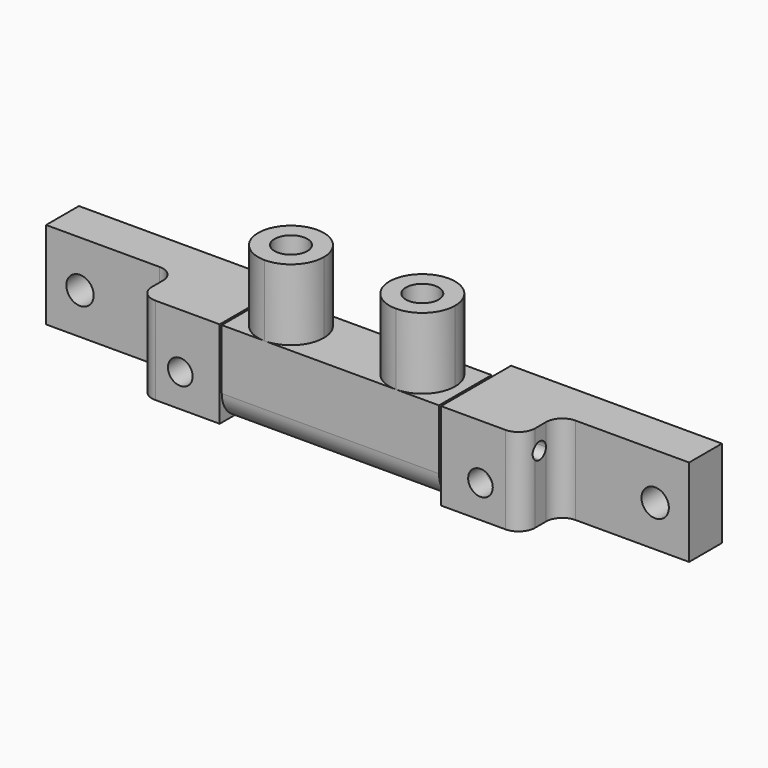
from build123d import *

# Parameters (mm, degrees)
F0_W     = 23.75
F0_H     = 3.5
F1_DEPTH = 16
F0_R     = 3
F2_DEPTH = 29
F3_R     = 2.25
F3_R_2   = 2.5
F4_DEPTH = 12.5
F5_R     = 3
F5_2_R   = 3
F7_DEPTH = 40
F8_R     = 5


with BuildPart() as f1:
    # F0 (on Top) → F1 (new body)
    with BuildSketch(Plane.XY):
        with Locations((-46.875, 6.25)):
            Rectangle(F0_W, F0_H)
        Polygon((-20.2244706452, -4), (-20.2244706452, 8), (-35, 8), (-35, 4.5), (-35, -4), align=None)
        Polygon((-35, 8), (-20.2244706452, 8), (-20.2244706452, 12), (-58.75, 12), (-58.75, 8), align=None)
    extrude(amount=F1_DEPTH)


with BuildPart() as f1b:
    # F0 (on Top) → F1, piece 2 (new body)
    with BuildSketch(Plane.XY):
        with BuildLine():
            ThreePointArc((-12, -4), (-18, 2.0000000001), (-11.9999999997, 8))
            Line((-11.9999999997, 8), (-19.8490470648, 8))
            Line((-19.8490470648, 8), (-19.8490470648, -4))
            Line((-19.8490470648, -4), (-12, -4))
        make_face()
        with BuildLine():
            ThreePointArc((-6, 2), (-7.7573593128, 6.242640687), (-11.9999999997, 8))
            ThreePointArc((-11.9999999997, 8), (-18, 2.0000000001), (-12, -4))
            ThreePointArc((-12, -4), (-7.7573593129, -2.2426406871), (-6, 2))
        make_face()
        with Locations((-12, 2)):
            Circle(F0_R, mode=Mode.SUBTRACT)
        with Locations((-12, 2)):
            Circle(F0_R)
        with BuildLine():
            ThreePointArc((12, -4), (6, 2.0000000207), (12.0000000413, 8))
            Line((12.0000000413, 8), (-11.9999999997, 8))
            ThreePointArc((-11.9999999997, 8), (-7.7573593128, 6.242640687), (-6, 2))
            ThreePointArc((-6, 2), (-7.7573593129, -2.2426406871), (-12, -4))
            Line((-12, -4), (12, -4))
        make_face()
        with BuildLine():
            ThreePointArc((18, 2), (17.8620020617, 3.2794263668), (17.4543560573, 4.5))
            ThreePointArc((17.4543560573, 4.5), (15.2403703666, 7.049752458), (12.0000000413, 8))
            ThreePointArc((12.0000000413, 8), (6, 2.0000000207), (12, -4))
            ThreePointArc((12, -4), (16.2426406871, -2.2426406871), (18, 2))
        make_face()
        with BuildLine():
            ThreePointArc((13.6583123952, 4.5), (14.6433820369, 3.4186371655), (15, 2))
            ThreePointArc((15, 2), (9.3566179631, 0.5813628345), (13.6583123952, 4.5))
        make_face(mode=Mode.SUBTRACT)
        with BuildLine():
            ThreePointArc((13.6583123952, 4.5), (9.3566179631, 0.5813628345), (15, 2))
            ThreePointArc((15, 2), (14.6433820369, 3.4186371655), (13.6583123952, 4.5))
        make_face()
        with BuildLine():
            ThreePointArc((12.0000000413, 8), (15.2403703666, 7.049752458), (17.4543560573, 4.5))
            ThreePointArc((17.4543560573, 4.5), (17.8620020617, 3.2794263668), (18, 2))
            ThreePointArc((18, 2), (16.2426406871, -2.2426406871), (12, -4))
            Line((12, -4), (19.8490470648, -4))
            Line((19.8490470648, -4), (19.8490470648, 8))
            Line((19.8490470648, 8), (12.0000000413, 8))
        make_face()
    extrude(amount=F1_DEPTH)

    # F0 (on Top) → F2 (join)
    with BuildSketch(Plane.XY):
        with BuildLine():
            ThreePointArc((-6, 2), (-7.7573593128, 6.242640687), (-11.9999999997, 8))
            ThreePointArc((-11.9999999997, 8), (-18, 2.0000000001), (-12, -4))
            ThreePointArc((-12, -4), (-7.7573593129, -2.2426406871), (-6, 2))
        make_face()
        with Locations((-12, 2)):
            Circle(F0_R, mode=Mode.SUBTRACT)
        with BuildLine():
            ThreePointArc((18, 2), (17.8620020617, 3.2794263668), (17.4543560573, 4.5))
            ThreePointArc((17.4543560573, 4.5), (15.2403703666, 7.049752458), (12.0000000413, 8))
            ThreePointArc((12.0000000413, 8), (6, 2.0000000207), (12, -4))
            ThreePointArc((12, -4), (16.2426406871, -2.2426406871), (18, 2))
        make_face()
        with BuildLine():
            ThreePointArc((13.6583123952, 4.5), (14.6433820369, 3.4186371655), (15, 2))
            ThreePointArc((15, 2), (9.3566179631, 0.5813628345), (13.6583123952, 4.5))
        make_face(mode=Mode.SUBTRACT)
    extrude(amount=F2_DEPTH)


with BuildPart() as f1c:
    # F0 (on Top) → F1, piece 3 (new body)
    with BuildSketch(Plane.XY):
        Polygon((35, 8), (20.2244706452, 8), (20.2244706452, -4), (35, -4), (35, 4.5), align=None)
        with Locations((46.875, 6.25)):
            Rectangle(F0_W, F0_H)
        Polygon((20.2244706452, 12), (20.2244706452, 8), (35, 8), (58.75, 8), (58.75, 12), align=None)
    extrude(amount=F1_DEPTH)


with BuildPart() as f4_tool:
    # F3 (on Front) → F4 (new body, symmetric)
    with BuildSketch(Plane.XZ):
        with Locations((-27.4271778762, 6)):
            Circle(F3_R)
        with Locations((27.4271778762, 6)):
            Circle(F3_R)
        with Locations((-52.55, 7.5)):
            Circle(F3_R_2)
        with Locations((52.55, 7.5)):
            Circle(F3_R_2)
    extrude(amount=F4_DEPTH, both=True)


with BuildPart() as f1_1:
    add(f1.part)

    # F4: cut by f4_tool
    add(f4_tool.part, mode=Mode.SUBTRACT)

    # F5
    f5_edges = [f1_1.edges().sort_by_distance(p)[0] for p in [
        (-35, -4, 8),
        (-35, 4.5, 8),
    ]]
    fillet(f5_edges, radius=F5_R)


with BuildPart() as f1c_1:
    add(f1c.part)

    # F4: cut by f4_tool
    add(f4_tool.part, mode=Mode.SUBTRACT)

    # F5#2
    f5_2_edges = [f1c_1.edges().sort_by_distance(p)[0] for p in [
        (35, 4.5, 8),
        (35, -4, 8),
    ]]
    fillet(f5_2_edges, radius=F5_2_R)


with BuildPart() as f7_tool:
    # F6 (on Right) → F7 (new body, symmetric)
    with BuildSketch(Plane.YZ):
        with BuildLine():
            ThreePointArc((0, 10.5), (1.0606601718, 10.9393398282), (1.5, 12))
            ThreePointArc((1.5, 12), (-1.0606601718, 13.0606601718), (0, 10.5))
        make_face()
    extrude(amount=F7_DEPTH, both=True)


with BuildPart() as f1_2:
    add(f1_1.part)

    # F7: cut by f7_tool
    add(f7_tool.part, mode=Mode.SUBTRACT)


with BuildPart() as f1b_1:
    add(f1b.part)

    # F7: cut by f7_tool
    add(f7_tool.part, mode=Mode.SUBTRACT)

    # F8
    f8_edges = [f1b_1.edges().sort_by_distance(p)[0] for p in [
        (0, -4, 0),
        (0, 8, 0),
    ]]
    fillet(f8_edges, radius=F8_R)


with BuildPart() as f1c_2:
    add(f1c_1.part)

    # F7: cut by f7_tool
    add(f7_tool.part, mode=Mode.SUBTRACT)


solid = Compound([f1_2.part, f1b_1.part, f1c_2.part])
